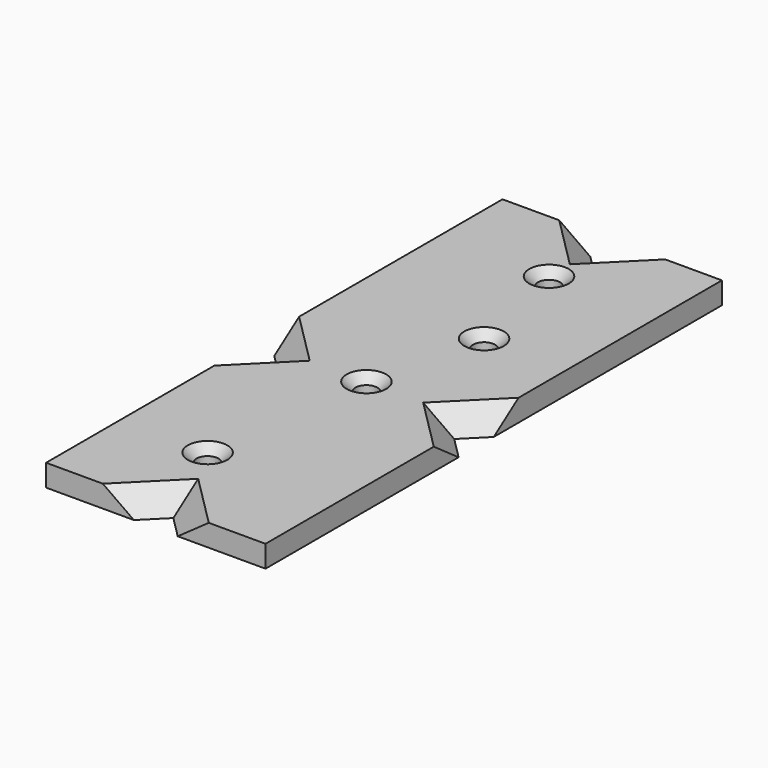
from build123d import *

# Parameters (mm, degrees)
F0_R     = 2.5
F1_DEPTH = 5
F2_SIZE  = 4.99999
F3_SIZE  = 2


# Not quite as in the source:
# - a fillet or chamfer is up to 0.001 mm smaller than in the source, because OpenCascade refuses the exact size


with BuildPart() as f1:
    # F0 (on Top) → F1 (new body)
    with BuildSketch(Plane.XY):
        Polygon((-5, 70), (-25, 70), (-25, 5), (-20, 0), (-25, -5), (-25, -60), (-5, -60), (0, -55), (5, -60), (25, -60), (25, -5), (20, 0), (25, 5), (25, 70), (5, 70), (0, 65), align=None)
        with Locations((-4.9999998882, -39)):
            Circle(F0_R, mode=Mode.SUBTRACT)
        Circle(F0_R, mode=Mode.SUBTRACT)
        with Locations((6, 26)):
            Circle(F0_R, mode=Mode.SUBTRACT)
        with Locations((0, 52)):
            Circle(F0_R, mode=Mode.SUBTRACT)
    extrude(amount=F1_DEPTH)

    # F2 (size 5 in the source; OpenCascade refuses exactly that, so slightly less here)
    f2_edges = [f1.edges().sort_by_distance(p)[0] for p in [
        (-2.5, 67.5, 5),
        (2.5, 67.5, 5),
        (22.5, 2.5, 5),
        (22.5, -2.5, 5),
        (-22.5, 2.5, 5),
        (-22.5, -2.5, 5),
        (-2.5, -57.5, 5),
        (2.5, -57.5, 5),
    ]]
    chamfer(f2_edges, length=F2_SIZE)

    # F3
    f3_edges = [f1.edges().sort_by_distance(p)[0] for p in [
        (-2.5, 52, 5),
        (3.5, 26, 5),
        (-7.5, -39, 5),
        (-2.5, 0, 5),
    ]]
    chamfer(f3_edges, length=F3_SIZE)


solid = f1.part
